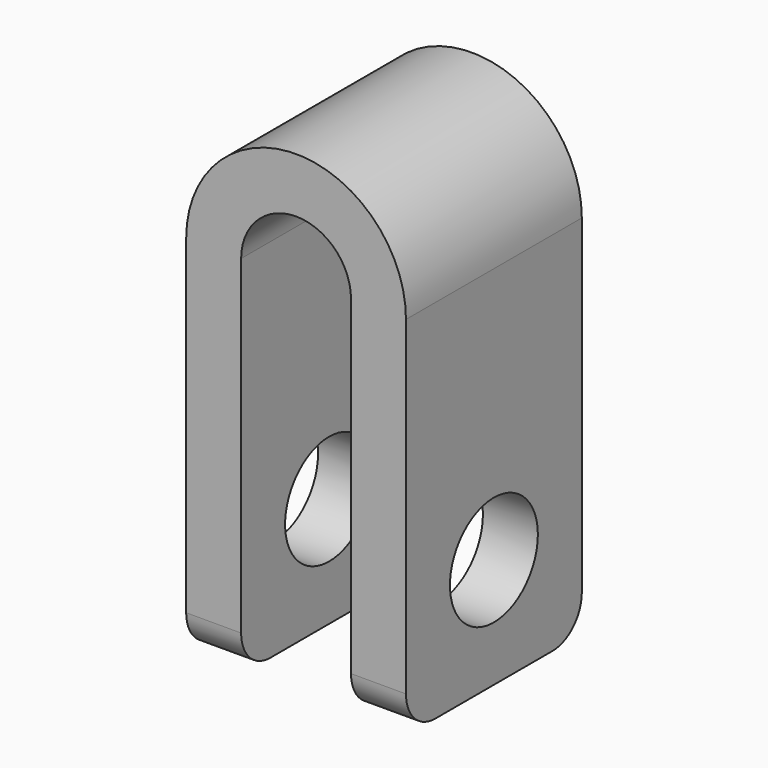
from build123d import *

# Parameters (mm, degrees)
F1_DEPTH = 6
F3_D     = 3
F4_R     = 1


# Not quite as in the source:
# - a feature names something its author has since deleted; it is built from what else it names


with BuildPart() as f1:
    # F0 (on Front) → F1 (new body)
    with BuildSketch(Plane.XZ):
        with BuildLine():
            Line((-1.5, -10), (-1.5, 0))
            ThreePointArc((-1.5, 0), (0, 1.5), (1.5, 0))
            Line((1.5, 0), (1.5, -10))
            Line((1.5, -10), (3, -10))
            Line((3, -10), (3, 0))
            ThreePointArc((3, 0), (0, 3), (-3, 0))
            Line((-3, 0), (-3, -10))
            Line((-3, -10), (-1.5, -10))
        make_face()
    extrude(amount=F1_DEPTH)

    # F3 (through all)
    with Locations(Plane(origin=(-3, 0, 0), x_dir=(0, -1, 0), z_dir=(-1, 0, 0))):
        with Locations((3, -7)):
            Hole(F3_D / 2)

    # F4
    f4_edges = [f1.edges().sort_by_distance(p)[0] for p in [
        (-2.25, -6, -10),
        (2.25, -6, -10),
        (2.25, 0, -10),
        (-2.25, 0, -10),
    ]]
    fillet(f4_edges, radius=F4_R)


solid = f1.part
